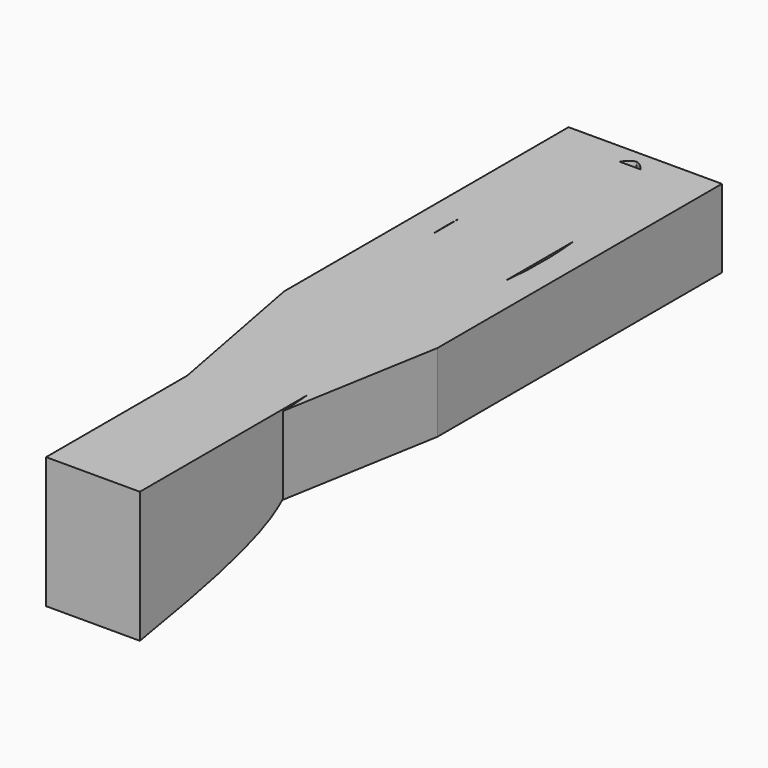
from build123d import *

# Parameters (mm, degrees)
F2_DEPTH = 42
F3_DEPTH = 50
F4_DEPTH = 35


with BuildPart() as f2:
    # F1 (on Right) → F2 (new body)
    with BuildSketch(Plane.YZ):
        with BuildLine():
            Line((150, 35), (-150, 35))
            Line((-150, 35), (-150, -23.7761443613))
            add(Edge.make_bspline(
                [(-150, -23.7761443613), (-114.4989336933, -17.6506601351), (-63.6066313007, -8.0329394516), (-65.3826376361, 27.3288233891), (48.3048096846, 13.9929555256), (115.32909223, 27.83807524), (150, 35)],
                knots=[0.0176256107, 0.0176256107, 0.0176256107, 0.0176256107, 0.2771319135, 0.4057749729, 0.6926140747, 1, 1, 1, 1], degree=3))
        make_face()
    extrude(amount=F2_DEPTH)

    # F0 (on Top) → F3 (cut)
    with BuildSketch(Plane.XY):
        with BuildLine():
            Line((-13.4228849784, 0), (0, -71.0220535528))
            add(Edge.make_bspline(
                [(0, -71.0220535528), (0, -48.0822075317), (15.7714172383, 2.9708873893), (-9.184915464, 68.9182100809), (10.146482255, 142.7383784786), (17.930894995, 151.4622155134)],
                knots=[0, 0, 0, 0, 0.2430856885, 0.5044652694, 0.7195950008, 0.7195950008, 0.7195950008, 0.7195950008], degree=3))
            add(Edge.make_bspline(
                [(21.4410424232, 153.6304205656), (20.2112647145, 153.6956795849), (19.0445034859, 152.9269522058), (17.930894995, 151.4622155134)],
                knots=[0.752832966, 0.752832966, 0.752832966, 0.752832966, 0.7890941529, 0.7890941529, 0.7890941529, 0.7890941529], degree=3))
            add(Edge.make_bspline(
                [(21.4410424232, 153.6304205656), (22.670820132, 153.6956795849), (23.8375813606, 152.9269522058), (24.9511898515, 151.4622155134)],
                knots=[0.752832966, 0.752832966, 0.752832966, 0.752832966, 0.7890941529, 0.7890941529, 0.7890941529, 0.7890941529], degree=3))
            add(Edge.make_bspline(
                [(42.8820848465, -71.0220535528), (42.8820848465, -48.0822075317), (27.1106676082, 2.9708873893), (52.0670003105, 68.9182100809), (32.7356025915, 142.7383784786), (24.9511898515, 151.4622155134)],
                knots=[0, 0, 0, 0, 0.2430856885, 0.5044652694, 0.7195950008, 0.7195950008, 0.7195950008, 0.7195950008], degree=3))
            Line((42.8820848465, -71.0220535528), (55.256780237, 0))
            Line((55.256780237, 0), (55.256780237, 159.2645645142))
            Line((55.256780237, 159.2645645142), (-13.4228849784, 159.2645645142))
            Line((-13.4228849784, 159.2645645142), (-13.4228849784, 0))
        make_face()
        with BuildLine():
            add(Edge.make_bspline(
                [(21.4410424232, 153.6304205656), (20.2112647145, 153.6956795849), (19.0445034859, 152.9269522058), (17.930894995, 151.4622155134)],
                knots=[0.752832966, 0.752832966, 0.752832966, 0.752832966, 0.7890941529, 0.7890941529, 0.7890941529, 0.7890941529], degree=3))
            add(Edge.make_bspline(
                [(17.930894995, 151.4622155134), (19.1336020212, 152.8100654344), (20.3137955765, 153.5706024186), (21.4410424232, 153.6304205656)],
                knots=[0.7195950008, 0.7195950008, 0.7195950008, 0.7195950008, 0.752832966, 0.752832966, 0.752832966, 0.752832966], degree=3))
        make_face()
        with BuildLine():
            add(Edge.make_bspline(
                [(21.4410424232, 153.6304205656), (22.670820132, 153.6956795849), (23.8375813606, 152.9269522058), (24.9511898515, 151.4622155134)],
                knots=[0.752832966, 0.752832966, 0.752832966, 0.752832966, 0.7890941529, 0.7890941529, 0.7890941529, 0.7890941529], degree=3))
            add(Edge.make_bspline(
                [(24.9511898515, 151.4622155134), (23.7484828253, 152.8100654344), (22.56828927, 153.5706024186), (21.4410424232, 153.6304205656)],
                knots=[0.7195950008, 0.7195950008, 0.7195950008, 0.7195950008, 0.752832966, 0.752832966, 0.752832966, 0.752832966], degree=3))
        make_face()
    extrude(amount=-F3_DEPTH, mode=Mode.SUBTRACT)

    # F0 (on Top) → F4 (join)
    with BuildSketch(Plane.XY):
        with BuildLine():
            Line((-13.4228849784, 0), (0, -71.0220535528))
            add(Edge.make_bspline(
                [(0, -71.0220535528), (0, -48.0822075317), (15.7714172383, 2.9708873893), (-9.184915464, 68.9182100809), (10.146482255, 142.7383784786), (17.930894995, 151.4622155134)],
                knots=[0, 0, 0, 0, 0.2430856885, 0.5044652694, 0.7195950008, 0.7195950008, 0.7195950008, 0.7195950008], degree=3))
            add(Edge.make_bspline(
                [(21.4410424232, 153.6304205656), (20.2112647145, 153.6956795849), (19.0445034859, 152.9269522058), (17.930894995, 151.4622155134)],
                knots=[0.752832966, 0.752832966, 0.752832966, 0.752832966, 0.7890941529, 0.7890941529, 0.7890941529, 0.7890941529], degree=3))
            add(Edge.make_bspline(
                [(21.4410424232, 153.6304205656), (22.670820132, 153.6956795849), (23.8375813606, 152.9269522058), (24.9511898515, 151.4622155134)],
                knots=[0.752832966, 0.752832966, 0.752832966, 0.752832966, 0.7890941529, 0.7890941529, 0.7890941529, 0.7890941529], degree=3))
            add(Edge.make_bspline(
                [(42.8820848465, -71.0220535528), (42.8820848465, -48.0822075317), (27.1106676082, 2.9708873893), (52.0670003105, 68.9182100809), (32.7356025915, 142.7383784786), (24.9511898515, 151.4622155134)],
                knots=[0, 0, 0, 0, 0.2430856885, 0.5044652694, 0.7195950008, 0.7195950008, 0.7195950008, 0.7195950008], degree=3))
            Line((42.8820848465, -71.0220535528), (55.256780237, 0))
            Line((55.256780237, 0), (55.256780237, 159.2645645142))
            Line((55.256780237, 159.2645645142), (-13.4228849784, 159.2645645142))
            Line((-13.4228849784, 159.2645645142), (-13.4228849784, 0))
        make_face()
        with BuildLine():
            add(Edge.make_bspline(
                [(21.4410424232, 153.6304205656), (20.2112647145, 153.6956795849), (19.0445034859, 152.9269522058), (17.930894995, 151.4622155134)],
                knots=[0.752832966, 0.752832966, 0.752832966, 0.752832966, 0.7890941529, 0.7890941529, 0.7890941529, 0.7890941529], degree=3))
            add(Edge.make_bspline(
                [(17.930894995, 151.4622155134), (19.1336020212, 152.8100654344), (20.3137955765, 153.5706024186), (21.4410424232, 153.6304205656)],
                knots=[0.7195950008, 0.7195950008, 0.7195950008, 0.7195950008, 0.752832966, 0.752832966, 0.752832966, 0.752832966], degree=3))
        make_face()
        with BuildLine():
            add(Edge.make_bspline(
                [(21.4410424232, 153.6304205656), (22.670820132, 153.6956795849), (23.8375813606, 152.9269522058), (24.9511898515, 151.4622155134)],
                knots=[0.752832966, 0.752832966, 0.752832966, 0.752832966, 0.7890941529, 0.7890941529, 0.7890941529, 0.7890941529], degree=3))
            add(Edge.make_bspline(
                [(24.9511898515, 151.4622155134), (23.7484828253, 152.8100654344), (22.56828927, 153.5706024186), (21.4410424232, 153.6304205656)],
                knots=[0.7195950008, 0.7195950008, 0.7195950008, 0.7195950008, 0.752832966, 0.752832966, 0.752832966, 0.752832966], degree=3))
        make_face()
    extrude(amount=F4_DEPTH)


solid = f2.part
